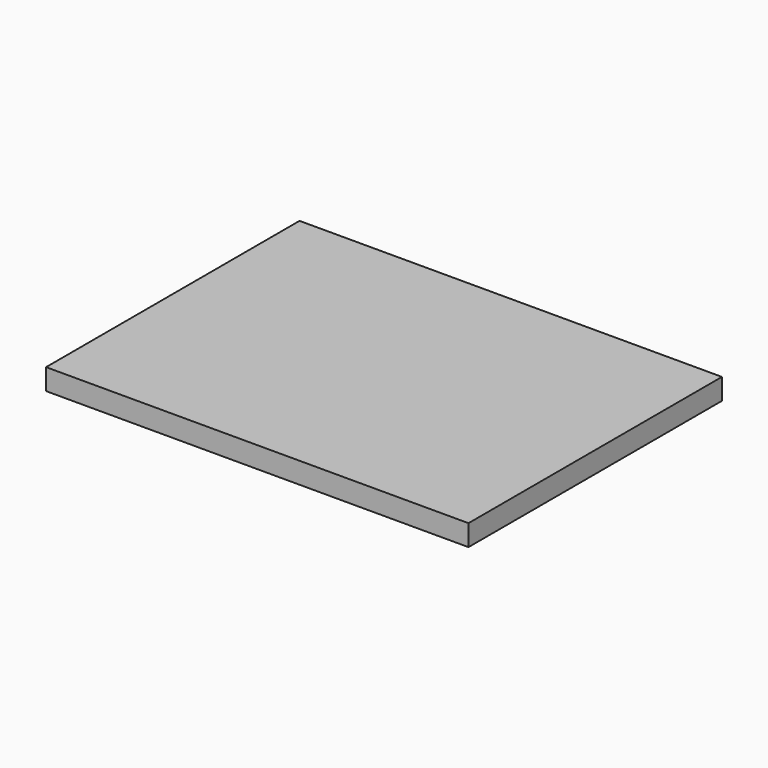
from build123d import *

# Parameters (mm, degrees)
F0_W     = 50.8
F0_H     = 38.1
F1_DEPTH = 2.54


# Not quite as in the source:
# - the program builds the solid bodies; features that only make, move or delete a surface that nothing else refers to are left out


with BuildPart() as f1:
    # F0 (on Top) → F1 (new body)
    with BuildSketch(Plane.XY):
        with Locations((25.4, 19.05)):
            Rectangle(F0_W, F0_H)
    extrude(amount=F1_DEPTH)


solid = f1.part
